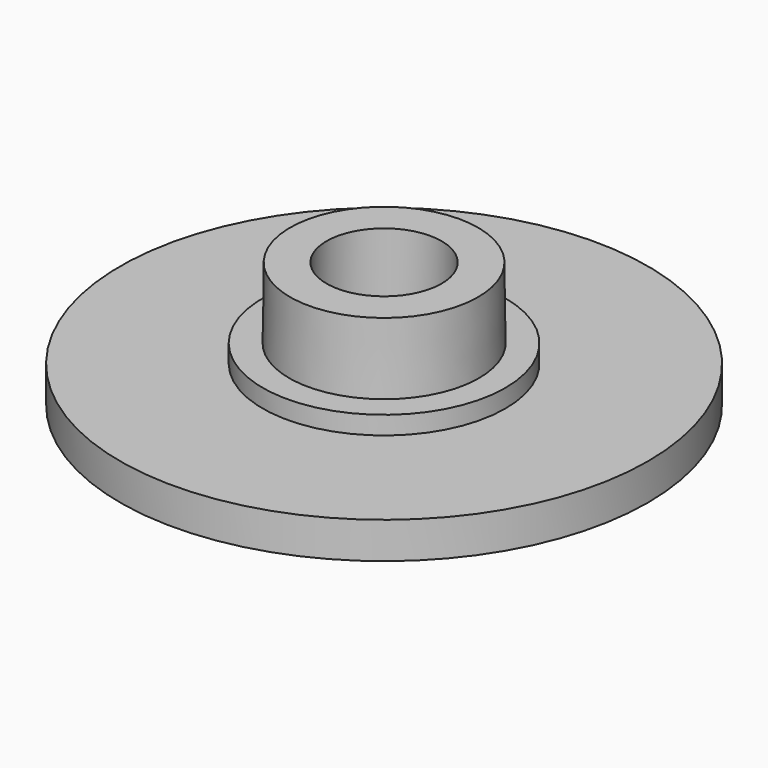
from build123d import *

# Parameters (mm, degrees)
F2_R     = 3.937
F2_R_2   = 2.667
F3_DEPTH = 2.794
F4_R     = 5.08
F5_DEPTH = 0.762
F6_R     = 11.049
F7_DEPTH = 1.524


with BuildPart() as f1:
    # F0 (on Right) → F1 (revolve)
    with BuildSketch(Plane.YZ):
        Polygon((2.4085466543, 2.8091624185), (2.4085466543, 0), (3.9751, 0), (3.937, 2.9743337072), (2.4085466543, 2.9743337072), align=None)
    revolve(axis=Axis((0, 0, 1.4871668536), (0, 0, 1)))



with BuildPart() as f3:
    # F2 (on Top) → F3 (new body)
    with BuildSketch(Plane.XY):
        Circle(F2_R)
        Circle(F2_R_2, mode=Mode.SUBTRACT)
    extrude(amount=F3_DEPTH)


with BuildPart() as f5:
    # F4 (on face) → F5 (new body)
    with BuildSketch(Plane(origin=(0, 0, 0), x_dir=(1, 0, 0), z_dir=(0, 0, -1))):
        Circle(F4_R)
    extrude(amount=F5_DEPTH)


with BuildPart() as f1_1:
    add(f1.part)

    add(f5.part)  # F7 merges F5
    # F6 (on face) → F7 (join)
    with BuildSketch(Plane(origin=(0, 0, -0.762), x_dir=(1, 0, 0), z_dir=(0, 0, -1))):
        Circle(F6_R)
    extrude(amount=F7_DEPTH)


solid = f1_1.part
